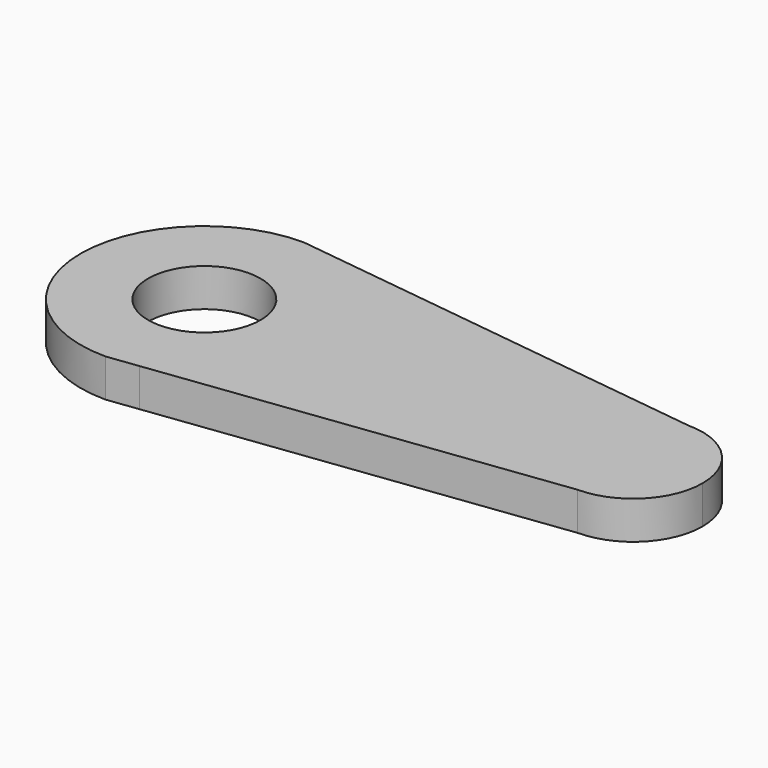
from build123d import *

# Parameters (mm, degrees)
F0_R     = 2.9612883312
F1_DEPTH = 2
F2_R     = 0.988841467
F3_DEPTH = 10


with BuildPart() as f1:
    # F0 (on Top) → F1 (new body)
    with BuildSketch(Plane.XY):
        with BuildLine():
            Line((1.6245851515, 6.3095047445), (0, 6.5152994586))
            ThreePointArc((0, 6.5152994586), (-6.5152994586, 0), (0, -6.5152994586))
            Line((0, -6.5152994586), (1.6245851515, -6.3095047445))
            ThreePointArc((1.6245851515, -6.3095047445), (5.1494555923, -3.9915202792), (6.5152994586, 0))
            ThreePointArc((6.5152994586, 0), (5.1494555923, 3.9915202792), (1.6245851515, 6.3095047445))
        make_face()
        Circle(F0_R, mode=Mode.SUBTRACT)
        with BuildLine():
            Line((22.574134171, 3.6557155928), (1.6245851515, 6.3095047445))
            ThreePointArc((1.6245851515, 6.3095047445), (5.1494555923, 3.9915202792), (6.5152994586, 0))
            ThreePointArc((6.5152994586, 0), (5.1494555923, -3.9915202792), (1.6245851515, -6.3095047445))
            Line((1.6245851515, -6.3095047445), (22.574134171, -3.6557155928))
            ThreePointArc((22.574134171, -3.6557155928), (18.9184185782, 0), (22.574134171, 3.6557155928))
        make_face()
        with BuildLine():
            ThreePointArc((26.2298497639, 0), (25.1591154568, 2.5849812858), (22.574134171, 3.6557155928))
            ThreePointArc((22.574134171, 3.6557155928), (18.9184185782, 0), (22.574134171, -3.6557155928))
            ThreePointArc((22.574134171, -3.6557155928), (25.1591154568, -2.5849812858), (26.2298497639, 0))
        make_face()
    extrude(amount=F1_DEPTH)

    # F2 (on face) → F3 (cut)
    with BuildSketch(Plane.XY.offset(2)):
        with Locations((22.574134171, 0)):
            Circle(F2_R)
    extrude(amount=F3_DEPTH, mode=Mode.SUBTRACT)


solid = f1.part
